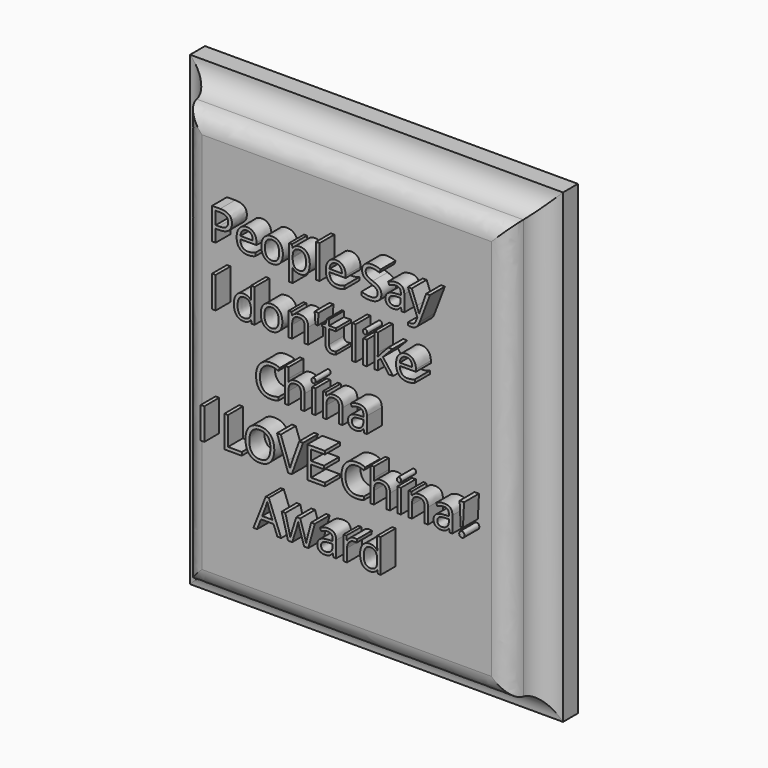
from build123d import *

# Parameters (mm, degrees)
F0_W         = 101.6
F0_H         = 127
F1_DEPTH     = 15.24
F2_W         = 101.6
F2_H         = 127
F2_W_2       = 88.9
F2_H_2       = 114.3
F3_DEPTH     = 10.16
F4_R         = 6.34999
F5_R         = 5.08
F6_TEXT_SIZE = 11.9580221229
F7_DEPTH     = 5.08


# Not quite as in the source:
# - a fillet or chamfer is up to 0.001 mm smaller than in the source, because OpenCascade refuses the exact size
# - Text() gives the source's letters only with a copy of the font that has no kerning and outlines rounded to 1/6400 em; it was checked with that copy


with BuildPart() as f1:
    # F0 (on Front) → F1 (new body)
    with BuildSketch(Plane.XZ):
        with Locations((-50.8, 63.5)):
            Rectangle(F0_W, F0_H)
    extrude(amount=F1_DEPTH)

    # F2 (on face) → F3 (cut)
    with BuildSketch(Plane.XZ.offset(15.24)):
        with Locations((-50.8, 63.5)):
            Rectangle(F2_W, F2_H)
        with Locations((-50.8, 63.5)):
            Rectangle(F2_W_2, F2_H_2, mode=Mode.SUBTRACT)
    extrude(amount=-F3_DEPTH, mode=Mode.SUBTRACT)

    # F4 (radius 6.35 in the source; OpenCascade refuses exactly that, so slightly less here)
    f4_edges = [f1.edges().sort_by_distance(p)[0] for p in [
        (-50.8, -5.08, 120.65),
        (-6.35, -5.08, 63.5),
        (-95.25, -5.08, 63.5),
        (-50.8, -5.08, 6.35),
    ]]
    fillet(f4_edges, radius=F4_R)

    # F5
    f5_edges = [f1.edges().sort_by_distance(p)[0] for p in [
        (-6.35, -15.24, 63.5),
        (-50.8, -15.24, 6.35),
        (-95.25, -15.24, 63.5),
        (-50.8, -15.24, 120.65),
    ]]
    fillet(f5_edges, radius=F5_R)

    # F6 (on face) → F7 (join)
    with BuildSketch(Plane.XZ.offset(15.24)):
        with Locations((-84.5935573633, 94.3309987458)):
            Text('People Say', F6_TEXT_SIZE, font='Open Sans', text_align=(TextAlign.LEFT, TextAlign.BOTTOM))
        with Locations((-84.5935573633, 78.0680886587)):
            Text("I don't like", F6_TEXT_SIZE, font='Open Sans', text_align=(TextAlign.LEFT, TextAlign.BOTTOM))
        with Locations((-72.1646881194, 61.8051785716)):
            Text('China', F6_TEXT_SIZE, font='Open Sans', text_align=(TextAlign.LEFT, TextAlign.BOTTOM))
        with Locations((-87.7007746743, 45.5422684845)):
            Text('I LOVE China!', F6_TEXT_SIZE, font='Open Sans', text_align=(TextAlign.LEFT, TextAlign.BOTTOM))
        with Locations((-72.1646881194, 29.2793583975)):
            Text('Award', F6_TEXT_SIZE, font='Open Sans', text_align=(TextAlign.LEFT, TextAlign.BOTTOM))
    extrude(amount=F7_DEPTH)


solid = f1.part
